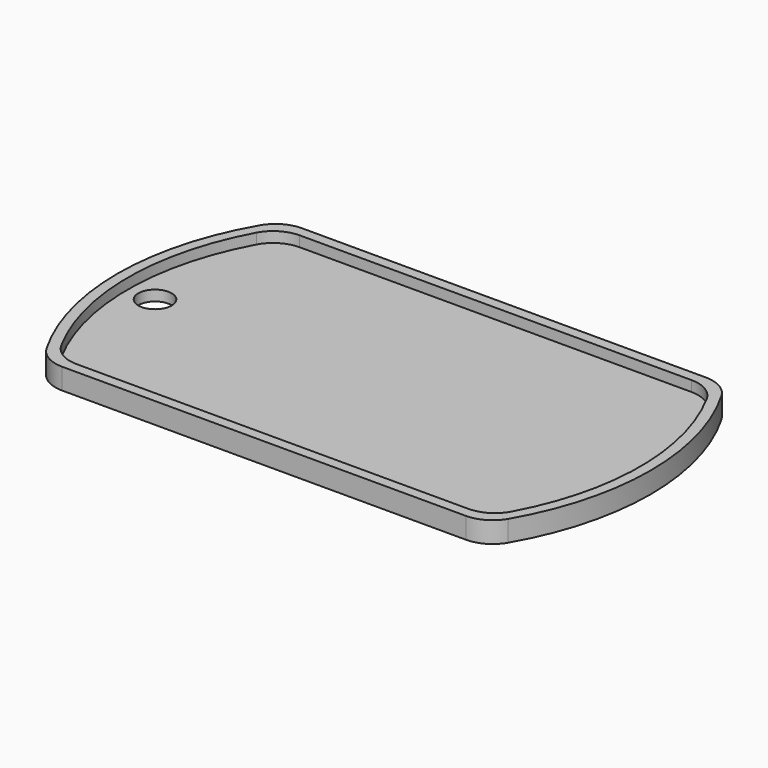
from build123d import *

# Parameters (mm, degrees)
F1_DEPTH = 1
F3_DEPTH = 1
F4_R     = 1.5875
F5_DEPTH = 1


# Not quite as in the source:
# - the program builds the solid bodies; features that only make, move or delete a surface that nothing else refers to are left out


with BuildPart() as f1:
    # F0 (on Top) → F1 (new body)
    with BuildSketch(Plane.XY):
        with BuildLine():
            ThreePointArc((-19.2474145991, 14.2875), (-20.8349145991, 13.862130657), (-21.9970452561, 12.7))
            ThreePointArc((-21.9970452561, 12.7), (-25.4, 0), (-21.9970452561, -12.7))
            ThreePointArc((-21.9970452561, -12.7), (-20.8349145991, -13.862130657), (-19.2474145991, -14.2875))
            Line((-19.2474145991, -14.2875), (19.2474145991, -14.2875))
            ThreePointArc((19.2474145991, -14.2875), (20.8349145991, -13.862130657), (21.9970452561, -12.7))
            ThreePointArc((21.9970452561, -12.7), (25.4, 0), (21.9970452561, 12.7))
            ThreePointArc((21.9970452561, 12.7), (20.8349145991, 13.862130657), (19.2474145991, 14.2875))
            Line((19.2474145991, 14.2875), (-19.2474145991, 14.2875))
        make_face()
    extrude(amount=F1_DEPTH)

    # F2 (on face) → F3 (join)
    with BuildSketch(Plane.XY.offset(1)):
        with BuildLine():
            Line((19.2474145991, 14.2875), (-19.2474145991, 14.2875))
            ThreePointArc((-19.2474145991, 14.2875), (-20.8349145991, 13.862130657), (-21.9970452561, 12.7))
            ThreePointArc((-21.9970452561, 12.7), (-25.4, 0), (-21.9970452561, -12.7))
            ThreePointArc((-21.9970452561, -12.7), (-20.8349145991, -13.862130657), (-19.2474145991, -14.2875))
            Line((-19.2474145991, -14.2875), (19.2474145991, -14.2875))
            ThreePointArc((19.2474145991, -14.2875), (20.8349145991, -13.862130657), (21.9970452561, -12.7))
            ThreePointArc((21.9970452561, -12.7), (25.4, 0), (21.9970452561, 12.7))
            ThreePointArc((21.9970452561, 12.7), (20.8349145991, 13.862130657), (19.2474145991, 14.2875))
        make_face()
        with BuildLine():
            ThreePointArc((-21.4526124879, 11.6252061249), (-20.2856017842, 12.8404540819), (-18.6611352482, 13.2875))
            Line((-18.6611352482, 13.2875), (18.6611352482, 13.2875))
            ThreePointArc((18.6611352482, 13.2875), (20.2856017842, 12.8404540819), (21.4526124879, 11.6252061249))
            ThreePointArc((21.4526124879, 11.6252061249), (24.4, 0), (21.4526124879, -11.6252061249))
            ThreePointArc((21.4526124879, -11.6252061249), (20.2856017842, -12.8404540819), (18.6611352482, -13.2875))
            Line((18.6611352482, -13.2875), (-18.6611352482, -13.2875))
            ThreePointArc((-18.6611352482, -13.2875), (-20.2856017842, -12.8404540819), (-21.4526124879, -11.6252061249))
            ThreePointArc((-21.4526124879, -11.6252061249), (-24.4, 0), (-21.4526124879, 11.6252061249))
        make_face(mode=Mode.SUBTRACT)
    extrude(amount=F3_DEPTH)

    # F4 (on face) → F5 (cut)
    with BuildSketch(Plane.XY.offset(1)):
        with Locations((-21.821282804, 0)):
            Circle(F4_R)
    extrude(amount=-F5_DEPTH, mode=Mode.SUBTRACT)


solid = f1.part
